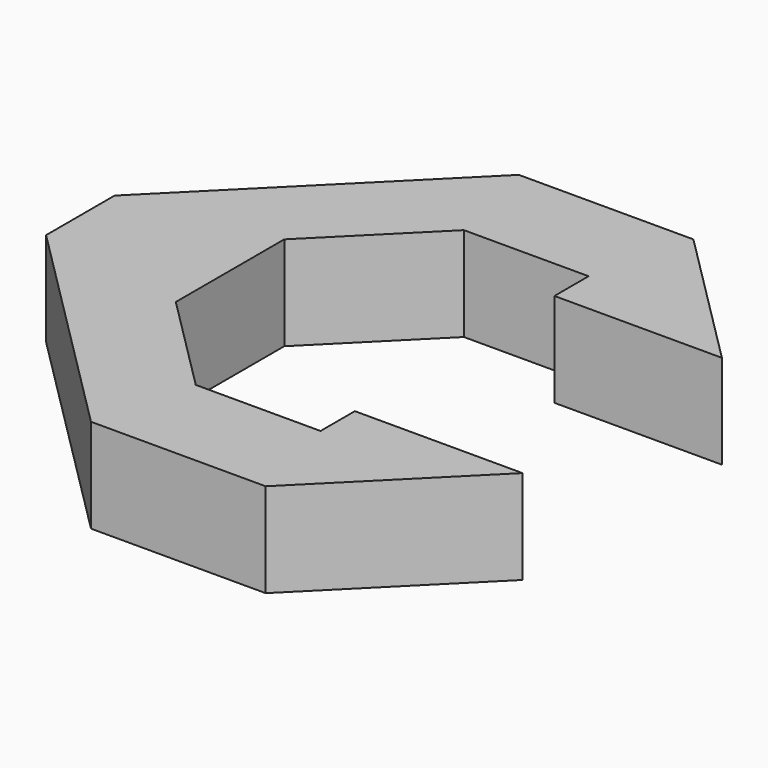
from build123d import *

# Parameters (mm, degrees)
F1_DEPTH    = 4.79011
F2_T1_DEPTH = 63.5787831049
F3_SIZE     = 5.08


# Not quite as in the source:
# - a fillet or chamfer that OpenCascade refuses, or shapes differently, is made with other operations: its cross-section is extruded or revolved along the edge and cut away or added


with BuildPart() as f1:
    # F0 (on Top) → F1 (new body)
    with BuildSketch(Plane.XY):
        Polygon((-50.0122293171, 11.8212979911), (-37.3122293171, 11.8212979911), (-37.3122293171, 19.0773104769), (-69.0622293171, 19.0773104769), (-69.0622293171, -8.1431020089), (-37.3122293171, -8.1431020089), (-37.3122293171, -0.8787020089), (-50.0122293171, -0.8787020089), (-50.0122293171, -3.0631020089), (-61.4422293171, -3.0631020089), (-61.4422293171, 13.9973104769), (-50.0122293171, 13.9973104769), align=None)
    extrude(amount=F1_DEPTH)

    # F2: chamfer of 11.43 on 4 edges, made by hand

    # F2_s2 → F2_t1 (cut)
    with BuildSketch(Plane.XY.offset(-29.3943365525)):
        Polygon((-57.6322293171, 19.0773104769), (-69.0622293171, 7.6473104769), (-69.0622293171, 19.0773104769), align=None)
        Polygon((-37.3122293171, 7.6473104769), (-48.7422293171, 19.0773104769), (-37.3122293171, 19.0773104769), align=None)
        Polygon((-48.7422293171, -8.1431020089), (-37.3122293171, 3.2868979911), (-37.3122293171, -8.1431020089), align=None)
        Polygon((-69.0622293171, 3.2868979911), (-57.6322293171, -8.1431020089), (-69.0622293171, -8.1431020089), align=None)
    extrude(amount=F2_T1_DEPTH, mode=Mode.SUBTRACT)

    # F3
    f3_edges = [f1.edges().sort_by_distance(p)[0] for p in [
        (-61.442229, 13.99731, 2.395055),
        (-61.442229, -3.063102, 2.395055),
    ]]
    chamfer(f3_edges, length=F3_SIZE)


solid = f1.part
